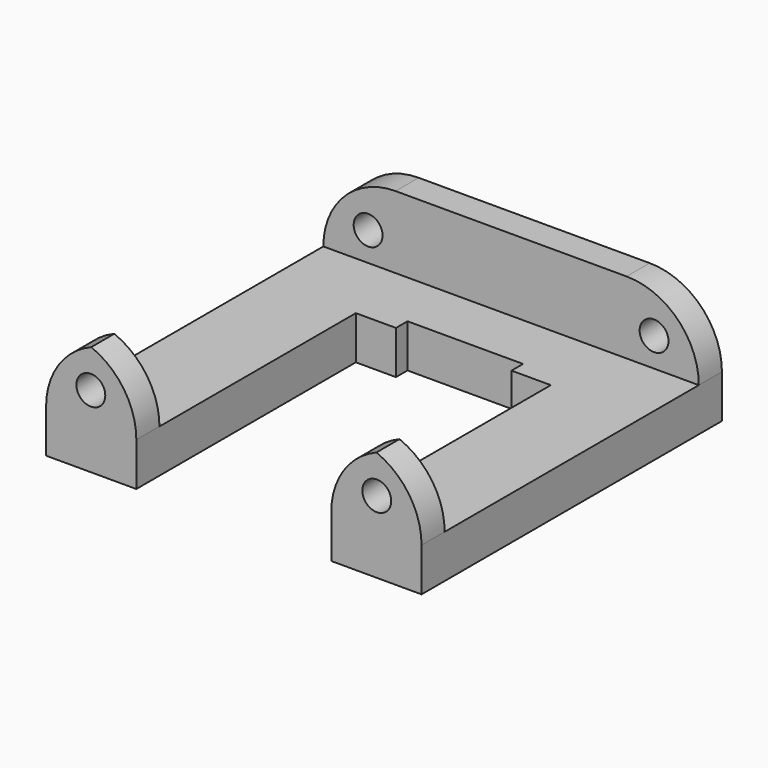
from build123d import *

# Parameters (mm, degrees)
F0_W        = 26
F0_H        = 2
F1_DEPTH    = 8
F0_W_2      = 6.25
F2_DEPTH    = 3
F3_T1_DEPTH = 27
F3_T3_DEPTH = 27
F4_R        = 1
F5_DEPTH    = 30


# Not quite as in the source:
# - a fillet or chamfer that OpenCascade refuses, or shapes differently, is made with other operations: its cross-section is extruded or revolved along the edge and cut away or added


with BuildPart() as f1:
    # F0 (on Top) → F1 (new body)
    with BuildSketch(Plane.XY):
        with Locations((0, 12)):
            Rectangle(F0_W, F0_H)
    extrude(amount=F1_DEPTH)



with BuildPart() as f1b:
    # F0 (on Top) → F1, piece 2 (new body)
    with BuildSketch(Plane.XY):
        with Locations((-9.875, -12)):
            Rectangle(F0_W_2, F0_H)
    extrude(amount=F1_DEPTH)


with BuildPart() as f1c:
    # F0 (on Top) → F1, piece 3 (new body)
    with BuildSketch(Plane.XY):
        with Locations((9.875, -12)):
            Rectangle(F0_W_2, F0_H)
    extrude(amount=F1_DEPTH)


with BuildPart() as f1_1:
    add(f1.part)

    add(f1b.part)  # F2 merges F1b

    add(f1c.part)  # F2 merges F1c
    # F0 (on Top) → F2 (join)
    with BuildSketch(Plane.XY):
        Polygon((6.75, -11), (13, -11), (13, 11), (-13, 11), (-13, -11), (-6.75, -11), (-6.75, 6), (-3.9725974202, 6), (-3.9725974202, 7), (4.0274025798, 7), (4.0274025798, 6), (6.75, 6), align=None)
    extrude(amount=F2_DEPTH)

    # F3: fillet of radius 5 on 6 edges, made by hand

    # F3_s2 → F3_t1 (cut)
    with BuildSketch(Plane.XZ.offset(-1.5)):
        with BuildLine():
            ThreePointArc((-8, 8), (-11.5355339059, 6.5355339059), (-13, 3))
            Line((-13, 3), (-13, 8))
            Line((-13, 8), (-8, 8))
        make_face()
        with BuildLine():
            ThreePointArc((-6.75, 3), (-8.2144660941, 6.5355339059), (-11.75, 8))
            Line((-11.75, 8), (-6.75, 8))
            Line((-6.75, 8), (-6.75, 3))
        make_face()
        with BuildLine():
            ThreePointArc((11.75, 8), (8.2144660941, 6.5355339059), (6.75, 3))
            Line((6.75, 3), (6.75, 8))
            Line((6.75, 8), (11.75, 8))
        make_face()
        with BuildLine():
            ThreePointArc((8, 8), (11.5355339059, 6.5355339059), (13, 3))
            Line((13, 3), (13, 8))
            Line((13, 8), (8, 8))
        make_face()
    extrude(amount=F3_T1_DEPTH, mode=Mode.SUBTRACT)

    # F3_s4 → F3_t3 (cut)
    with BuildSketch(Plane.XZ.offset(-25.5)):
        with BuildLine():
            ThreePointArc((8, 8), (11.5355339059, 6.5355339059), (13, 3))
            Line((13, 3), (13, 8))
            Line((13, 8), (8, 8))
        make_face()
        with BuildLine():
            ThreePointArc((-13, 3), (-11.5355339059, 6.5355339059), (-8, 8))
            Line((-8, 8), (-13, 8))
            Line((-13, 8), (-13, 3))
        make_face()
    extrude(amount=F3_T3_DEPTH, mode=Mode.SUBTRACT)

    # F4 (on face) → F5 (cut)
    with BuildSketch(Plane.XZ.offset(13)):
        with Locations((-9.9, 5)):
            Circle(F4_R)
        with Locations((9.9, 5)):
            Circle(F4_R)
    extrude(amount=-F5_DEPTH, mode=Mode.SUBTRACT)


solid = f1_1.part
